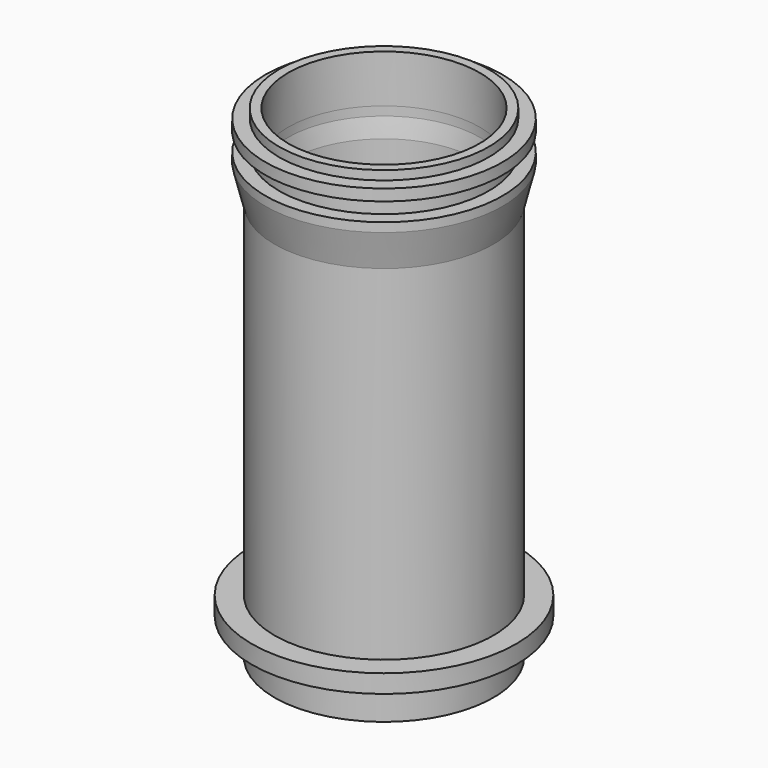
from build123d import *

# Parameters (mm, degrees)
F2_S5_R     = 16.67002
F2_T6_DEPTH = 26


# Not quite as in the source:
# - a fillet or chamfer that OpenCascade refuses, or shapes differently, is made with other operations: its cross-section is extruded or revolved along the edge and cut away or added


with BuildPart() as f1:
    # F0 (on Front) → F1 (revolve)
    with BuildSketch(Plane.XZ):
        Polygon((-17.7118646965, 0), (-16.1243646965, 1.5875), (-16.1243646965, 75.80376), (-16.67002, 75.80376), (-16.67002, 84.1375), (-18.25752, 84.1375), (-18.25752, 82.55), (-20.6375, 82.55), (-20.6375, 80.56626), (-18.2626, 80.56626), (-18.2626, 77.39126), (-20.6375, 77.39126), (-20.6375, 75.80376), (-19.05, 69.45376), (-19.05, 9.525), (-23.02002, 9.525), (-23.02002, 6.35), (-19.05, 6.35), (-19.05, 0), align=None)
    revolve(axis=Axis((0, 0, 38.1), (0, 0, 1)))

    # F2: chamfer of 0.8128 x 4.7625 on 1 edges, made by hand


with BuildPart() as f2_tool2:
    # F2_s3 → F2_t4 (revolve)
    with BuildSketch(Plane.XZ):
        Polygon((-16.1243646965, 71.04126), (-16.9371646965, 75.80376), (-16.1243646965, 75.80376), align=None)
    revolve(axis=Axis((0, 0, 75.80376), (0, 0, 1)))

    # F2_s5 → F2_t6 (intersect, symmetric)
    with BuildSketch(Plane.XY.offset(73.4)):
        Circle(F2_S5_R)
    extrude(amount=F2_T6_DEPTH, both=True, mode=Mode.INTERSECT)


with BuildPart() as f1_1:
    add(f1.part)

    # F2_t1: cut F2_tool2
    add(f2_tool2.part, mode=Mode.SUBTRACT)


solid = f1_1.part
